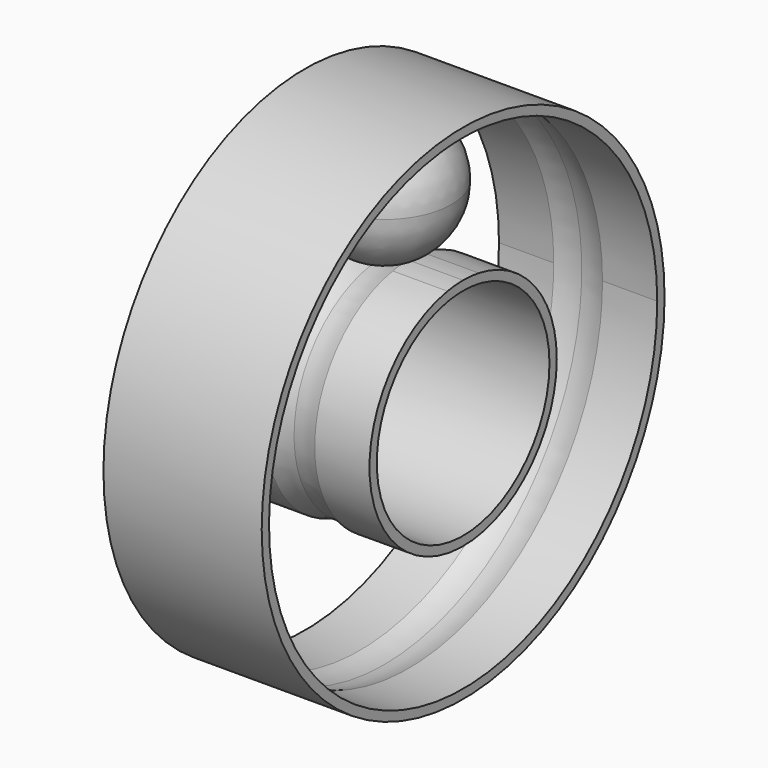
from build123d import *

# Parameters (mm, degrees)
F0_R     = 7.5
F1_DEPTH = 5.5
F0_R_2   = 17.5


with BuildPart() as f1:
    # F0 (on Right) → F1 (new body, symmetric)
    with BuildSketch(Plane.YZ):
        with BuildLine():
            ThreePointArc((-1.362401, 8.020105), (-5.248576, -6.215358), (8.135, 0))
            ThreePointArc((8.135, 0), (6.215358, 5.248576), (1.362401, 8.020105))
            ThreePointArc((1.362401, 8.020105), (0, 7.817523), (-1.362401, 8.020105))
        make_face()
        Circle(F0_R, mode=Mode.SUBTRACT)
        with BuildLine():
            ThreePointArc((-1.362401, 8.020105), (0, 7.817523), (1.362401, 8.020105))
            ThreePointArc((1.362401, 8.020105), (0.683619, 8.106225), (0, 8.135))
            ThreePointArc((0, 8.135), (-0.683619, 8.106225), (-1.362401, 8.020105))
        make_face()
    extrude(amount=F1_DEPTH, both=True)


with BuildPart() as f1b:
    # F0 (on Right) → F1, piece 2 (new body, symmetric)
    with BuildSketch(Plane.YZ):
        Circle(F0_R_2)
        with BuildLine():
            ThreePointArc((16.865, 0), (-11.209021, -12.601034), (-1.965248, 16.750105))
            ThreePointArc((-1.965248, 16.750105), (0, 17.182477), (1.965248, 16.750105))
            ThreePointArc((1.965248, 16.750105), (12.601034, 11.209021), (16.865, 0))
        make_face(mode=Mode.SUBTRACT)
        with BuildLine():
            ThreePointArc((1.965248, 16.750105), (0, 17.182477), (-1.965248, 16.750105))
            ThreePointArc((-1.965248, 16.750105), (-0.984302, 16.836252), (0, 16.865))
            ThreePointArc((0, 16.865), (0.984302, 16.836252), (1.965248, 16.750105))
        make_face()
    extrude(amount=F1_DEPTH, both=True)


with BuildPart() as f3_tool:
    # F2 (on Front) → F3 (revolve)
    with BuildSketch(Plane.XZ):
        with BuildLine():
            ThreePointArc((4.682477, 12.499975), (3.311011, 15.810986), (0, 17.182452))
            Line((0, 17.182452), (0, 12.499975))
            Line((0, 12.499975), (0, 7.817498))
            ThreePointArc((0, 7.817498), (3.311011, 9.188964), (4.682477, 12.499975))
        make_face()
        with BuildLine():
            Line((0, 12.499975), (0, 17.182452))
            ThreePointArc((0, 17.182452), (-4.682477, 12.499975), (0, 7.817498))
            Line((0, 7.817498), (0, 12.499975))
        make_face()
    revolve(axis=Axis((0, 0, 0), (-1, 0, 0)))


with BuildPart() as f1_1:
    add(f1.part)

    # F3: cut by f3_tool
    add(f3_tool.part, mode=Mode.SUBTRACT)


with BuildPart() as f1b_1:
    add(f1b.part)

    # F3: cut by f3_tool
    add(f3_tool.part, mode=Mode.SUBTRACT)


with BuildPart() as f4:
    # F0 (on Right) → F4 (revolve)
    with BuildSketch(Plane.YZ):
        with BuildLine():
            ThreePointArc((0, 8.135), (0.683619, 8.106225), (1.362401, 8.020105))
            ThreePointArc((1.362401, 8.020105), (3.761981, 9.711974), (4.682477, 12.5))
            ThreePointArc((4.682477, 12.5), (3.945112, 15.022238), (1.965248, 16.750105))
            ThreePointArc((1.965248, 16.750105), (0.984302, 16.836252), (0, 16.865))
            Line((0, 16.865), (0, 12.5))
            Line((0, 12.5), (0, 8.135))
        make_face()
    revolve(axis=Axis((0, 0, 14.6825), (0, 0, 1)))


solid = Compound([f1_1.part, f1b_1.part, f4.part])
